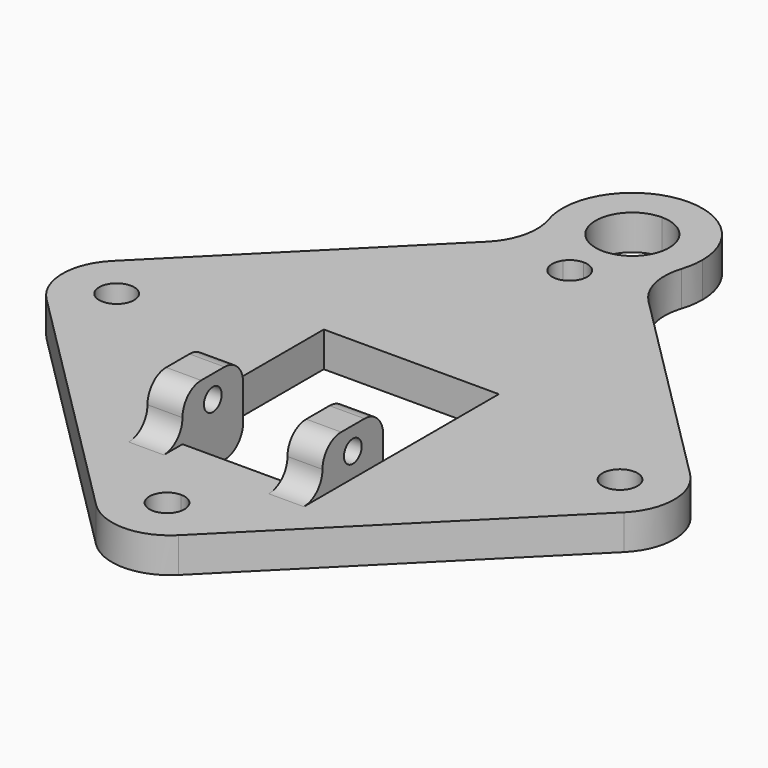
from build123d import *

# Parameters (mm, degrees)
F1_DEPTH = 3
F2_R     = 5
F0_W     = 3
F0_H     = 6.5
F3_DEPTH = 7
F4_R     = 0.95
F5_DEPTH = 25
F6_R     = 1.99999


# Not quite as in the source:
# - a fillet or chamfer is up to 0.001 mm smaller than in the source, because OpenCascade refuses the exact size
# - a feature names something its author has since deleted; it is built from what else it names


with BuildPart() as f1:
    # F0 (on Top) → F1 (new body)
    with BuildSketch(Plane.XY):
        with BuildLine():
            Line((-23.06675, 0), (-28.2842712475, 0))
            Line((-28.2842712475, 0), (0, -28.2842712475))
            Line((0, -28.2842712475), (0, -23.0667636524))
            ThreePointArc((0, -23.0667636524), (-1.5, -21.5667636524), (0, -20.0667636524))
            Line((0, -20.0667636524), (0, -14.2842712475))
            Line((0, -14.2842712475), (-4.5, -14.2842712475))
            Line((-4.5, -14.2842712475), (-7.5, -14.2842712475))
            Line((-7.5, -14.2842712475), (-7.5, -7.7842712475))
            Line((-7.5, -7.7842712475), (-7.5, 0))
            Line((-7.5, 0), (-20.06675, 0))
            ThreePointArc((-20.06675, 0), (-21.56675, -1.5), (-23.06675, 0))
        make_face()
        with BuildLine():
            Line((0, -23.0667636524), (0, -28.2842712475))
            Line((0, -28.2842712475), (28.2842712475, 0))
            Line((28.2842712475, 0), (23.06675, 0))
            ThreePointArc((23.06675, 0), (21.56675, -1.5), (20.06675, 0))
            Line((20.06675, 0), (7.5, 0))
            Line((7.5, 0), (7.5, -7.7842712475))
            Line((7.5, -7.7842712475), (7.5, -14.2842712475))
            Line((7.5, -14.2842712475), (4.5, -14.2842712475))
            Line((4.5, -14.2842712475), (0, -14.2842712475))
            Line((0, -14.2842712475), (0, -20.0667636524))
            ThreePointArc((0, -20.0667636524), (1.0606601718, -20.5061034806), (1.5, -21.5667636524))
            ThreePointArc((1.5, -21.5667636524), (1.0606601718, -22.6274238242), (0, -23.0667636524))
        make_face()
        with BuildLine():
            Line((-4.2426406871, 24.0416305603), (-28.2842712475, 0))
            Line((-28.2842712475, 0), (-23.06675, 0))
            ThreePointArc((-23.06675, 0), (-21.56675, 1.5), (-20.06675, 0))
            Line((-20.06675, 0), (-7.5, 0))
            Line((-7.5, 0), (-7.5, 4.6038874425))
            Line((-7.5, 4.6038874425), (0, 4.6038874425))
            Line((0, 4.6038874425), (0, 20.0667636524))
            ThreePointArc((0, 20.0667636524), (-1.3266484173, 20.8667608118), (-1.2382102141, 22.4134250167))
            ThreePointArc((-1.2382102141, 22.4134250167), (-2.8587925726, 23.0091120056), (-4.2426406871, 24.0416305603))
        make_face()
        with BuildLine():
            ThreePointArc((0, 34.2842712475), (-5.5432771951, 30.5803718417), (-4.2426406871, 24.0416305603))
            Line((-4.2426406871, 24.0416305603), (-2.2273863607, 26.0568848867))
            ThreePointArc((-2.2273863607, 26.0568848867), (-2.9102205274, 29.4897240594), (0, 31.4342712475))
            Line((0, 31.4342712475), (0, 34.2842712475))
        make_face()
        with BuildLine():
            Line((-2.2273863607, 26.0568848867), (-4.2426406871, 24.0416305603))
            ThreePointArc((-4.2426406871, 24.0416305603), (-2.8587925726, 23.0091120056), (-1.2382102141, 22.4134250167))
            ThreePointArc((-1.2382102141, 22.4134250167), (-0.7000028406, 22.8934120697), (0, 23.0667636524))
            Line((0, 23.0667636524), (0, 25.1342712475))
            ThreePointArc((0, 25.1342712475), (-1.205452812, 25.3740507201), (-2.2273863607, 26.0568848867))
        make_face()
        with BuildLine():
            ThreePointArc((6, 28.2842712475), (4.2426406871, 32.5269119346), (0, 34.2842712475))
            Line((0, 34.2842712475), (0, 31.4342712475))
            ThreePointArc((0, 31.4342712475), (2.2273863607, 30.5116576082), (3.15, 28.2842712475))
            ThreePointArc((3.15, 28.2842712475), (2.9102205274, 27.0788184355), (2.2273863607, 26.0568848867))
            Line((2.2273863607, 26.0568848867), (4.2426406871, 24.0416305603))
            ThreePointArc((4.2426406871, 24.0416305603), (5.5432771951, 25.9881706533), (6, 28.2842712475))
        make_face()
        with BuildLine():
            ThreePointArc((1.2382102141, 22.4134250167), (2.8587925726, 23.0091120056), (4.2426406871, 24.0416305603))
            Line((4.2426406871, 24.0416305603), (2.2273863607, 26.0568848867))
            ThreePointArc((2.2273863607, 26.0568848867), (1.2054528119, 25.3740507201), (0, 25.1342712475))
            Line((0, 25.1342712475), (0, 23.0667636524))
            ThreePointArc((0, 23.0667636524), (0.7000028406, 22.8934120697), (1.2382102141, 22.4134250167))
        make_face()
        with BuildLine():
            Line((23.06675, 0), (28.2842712475, 0))
            Line((28.2842712475, 0), (4.2426406871, 24.0416305603))
            ThreePointArc((4.2426406871, 24.0416305603), (2.8587925726, 23.0091120056), (1.2382102141, 22.4134250167))
            ThreePointArc((1.2382102141, 22.4134250167), (1.4330588476, 22.0098689891), (1.5, 21.5667636524))
            ThreePointArc((1.5, 21.5667636524), (1.0606601718, 20.5061034806), (0, 20.0667636524))
            Line((0, 20.0667636524), (0, 4.6038874425))
            Line((0, 4.6038874425), (7.5, 4.6038874425))
            Line((7.5, 4.6038874425), (7.5, 0))
            Line((7.5, 0), (20.06675, 0))
            ThreePointArc((20.06675, 0), (21.56675, 1.5), (23.06675, 0))
        make_face()
    extrude(amount=F1_DEPTH)

    # F2
    f2_edges = [f1.edges().sort_by_distance(p)[0] for p in [
        (-28.284271, 0, 1.5),
        (28.284271, 0, 1.5),
        (0, -28.284271, 1.5),
        (4.242641, 24.041631, 1.5),
        (-4.242641, 24.041631, 1.5),
    ]]
    fillet(f2_edges, radius=F2_R)

    # F0 (on Top) → F3 (join)
    with BuildSketch(Plane.XY):
        with Locations((-6, -11.0342712475)):
            Rectangle(F0_W, F0_H)
        with Locations((6, -11.0342712475)):
            Rectangle(F0_W, F0_H)
    extrude(amount=F3_DEPTH)

    # F4 (on face) → F5 (cut)
    with BuildSketch(Plane(origin=(-7.5, 0, 0), x_dir=(0, -1, 0), z_dir=(-1, 0, 0))):
        with Locations((11.0342712475, 5.05)):
            Circle(F4_R)
    extrude(amount=-F5_DEPTH, mode=Mode.SUBTRACT)

    # F6 (radius 2 in the source; OpenCascade refuses exactly that, so slightly less here)
    f6_edges = [f1.edges().sort_by_distance(p)[0] for p in [
        (-6, -14.284271, 7),
        (-6, -14.284271, 3),
        (-6, -7.784271, 7),
        (-6, -7.784271, 0),
        (6, -7.784271, 0),
        (6, -14.284271, 3),
        (6, -14.284271, 7),
        (6, -7.784271, 7),
    ]]
    fillet(f6_edges, radius=F6_R)


solid = f1.part
